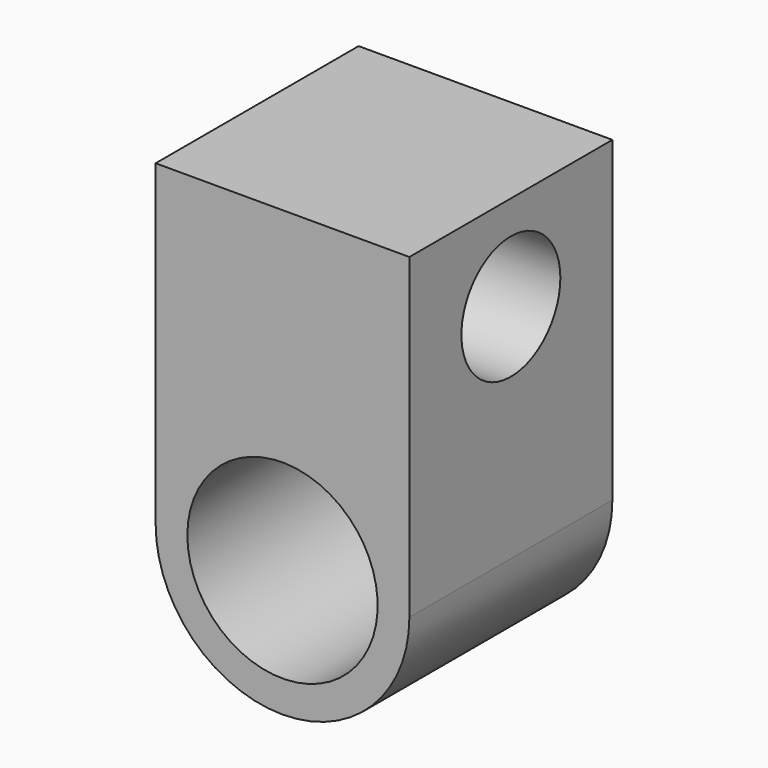
from build123d import *

# Parameters (mm, degrees)
F0_W          = 40
F0_H          = 70
F1_DEPTH      = 20
F1_DEPTH_BACK = 20
F3_D          = 19.5
F5_D          = 30
F6_R          = 19.99999


# Not quite as in the source:
# - a fillet or chamfer is up to 0.001 mm smaller than in the source, because OpenCascade refuses the exact size


with BuildPart() as f1:
    # F0 (on Front) → F1 (new body, two sides)
    with BuildSketch(Plane.XZ) as f1_sk:
        Rectangle(F0_W, F0_H)
    extrude(amount=F1_DEPTH)
    extrude(f1_sk.sketch, amount=-F1_DEPTH_BACK)

    # F3 (through all)
    with Locations(Plane(origin=(-20, 0, 0), x_dir=(0, -1, 0), z_dir=(-1, 0, 0))):
        with Locations((0, 20)):
            Hole(F3_D / 2)

    # F5 (through all)
    with Locations(Plane.XZ.offset(20)):
        with Locations((0, -15)):
            Hole(F5_D / 2)

    # F6 (radius 20 in the source; OpenCascade refuses exactly that, so slightly less here)
    f6_edges = [f1.edges().sort_by_distance(p)[0] for p in [
        (20, 0, -35),
        (-20, 0, -35),
    ]]
    fillet(f6_edges, radius=F6_R)


solid = f1.part
